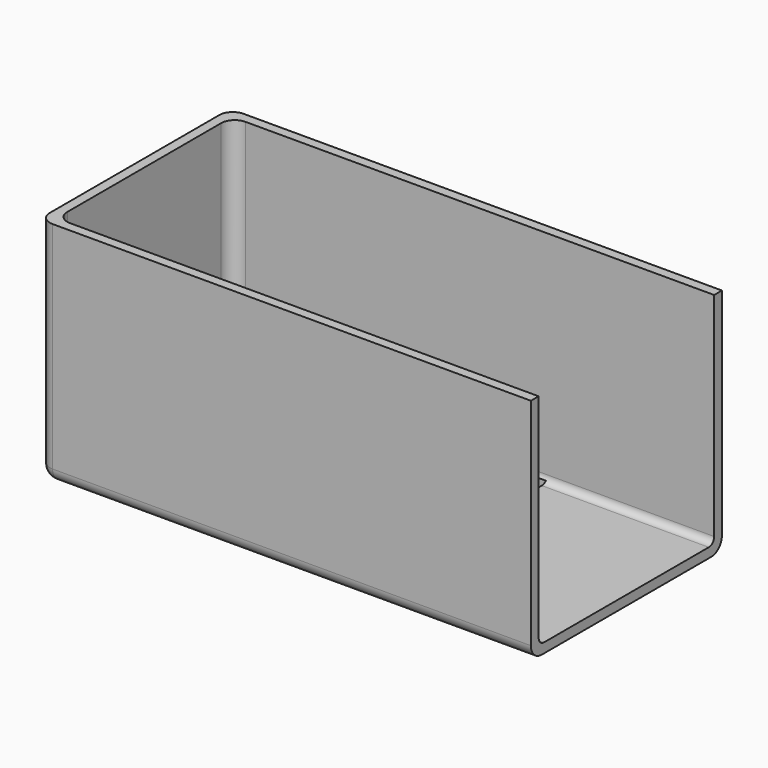
from build123d import *

# Parameters (mm, degrees)
F0_W         = 74.44
F0_H         = 35.44
F1_DEPTH     = 34
F2_T         = -1.44
F3_DEPTH     = 1.44
F4_R         = 2
F5_R         = 2
F6_W         = 22
F6_H         = 2
F7_DEPTH     = 1.441
F8_T1_DEPTH  = 28.56
F8_T6_DEPTH  = 69.56
F8_T12_DEPTH = 69.56
F8_T18_DEPTH = 69.56
F8_T25_DEPTH = 69.56
F8_T31_DEPTH = 69.56
F8_T35_ANGLE = 90
F8_T37_ANGLE = 90
F8_T41_DEPTH = 69.56
F8_T47_DEPTH = 69.56
F8_T53_DEPTH = 69.56
F8_T60_DEPTH = 69.56
F8_T66_DEPTH = 69.56


# Not quite as in the source:
# - a fillet or chamfer that OpenCascade refuses, or shapes differently, is made with other operations: its cross-section is extruded or revolved along the edge and cut away or added


with BuildPart() as f1:
    # F0 (on Top) → F1 (new body)
    with BuildSketch(Plane.XY):
        Rectangle(F0_W, F0_H)
    extrude(amount=F1_DEPTH)

    # F2
    f2_openings = [f1.faces().sort_by_distance(p)[0] for p in [
        (0, 0, 34),
    ]]
    offset(amount=F2_T, openings=f2_openings)

    # F3 (cut): a face of the model
    f3_faces = [f1.faces().sort_by_distance(p)[0] for p in [
        (37.22, 0, 17),
    ]]
    extrude(f3_faces, amount=-F3_DEPTH, mode=Mode.SUBTRACT)

    # F4
    f4_edges = [f1.edges().sort_by_distance(p)[0] for p in [
        (-35.78, -16.28, 17.72),
        (-35.78, 16.28, 17.72),
        (-37.22, 17.72, 17),
        (-37.22, -17.72, 17),
    ]]
    fillet(f4_edges, radius=F4_R)

    # F5
    f5_edges = [f1.edges().sort_by_distance(p)[0] for p in [
        (-37.22, 0, 0),
        (0.28, -17.72, 0),
        (0.28, 17.72, 0),
    ]]
    fillet(f5_edges, radius=F5_R)

    # F6 (on face) → F7 (cut, through all)
    with BuildSketch(Plane.XY.offset(1.44)):
        with Locations((0, 15.03)):
            Rectangle(F6_W, F6_H)
        with Locations((0, -15.03)):
            Rectangle(F6_W, F6_H)
    extrude(amount=-F7_DEPTH, mode=Mode.SUBTRACT)

    # F8: fillet of radius 1 on 1 edges, made by hand

    # F8_s2 → F8_t1 (join)
    with BuildSketch(Plane.XZ.offset(-14.28)):
        with BuildLine():
            ThreePointArc((-35.78, 2.44), (-35.4871067812, 1.7328932188), (-34.78, 1.44))
            Line((-34.78, 1.44), (-35.78, 1.44))
            Line((-35.78, 1.44), (-35.78, 2.44))
        make_face()
    extrude(amount=F8_T1_DEPTH)


with BuildPart() as f8_tool4:
    # F8_s5 → F8_t6 (new body)
    with BuildSketch(Plane.YZ.offset(-33.78)):
        with BuildLine():
            ThreePointArc((-16.28, 2.44), (-15.9871067812, 1.7328932188), (-15.28, 1.44))
            Line((-15.28, 1.44), (-16.28, 1.44))
            Line((-16.28, 1.44), (-16.28, 2.44))
        make_face()
    extrude(amount=F8_T6_DEPTH)

    split(bisect_by=Plane.YZ.offset(-11), keep=Keep.BOTTOM)

    split(bisect_by=Plane.XZ.offset(16.03), keep=Keep.TOP)


with BuildPart() as f1_1:
    add(f1.part)

    # F8_t3: union F8_tool4
    add(f8_tool4.part)


with BuildPart() as f8_tool10:
    # F8_s11 → F8_t12 (new body)
    with BuildSketch(Plane.YZ.offset(-33.78)):
        with BuildLine():
            ThreePointArc((-16.28, 2.44), (-15.9871067812, 1.7328932188), (-15.28, 1.44))
            Line((-15.28, 1.44), (-16.28, 1.44))
            Line((-16.28, 1.44), (-16.28, 2.44))
        make_face()
    extrude(amount=F8_T12_DEPTH)

    split(bisect_by=Plane.YZ.offset(-11), keep=Keep.BOTTOM)

    split(bisect_by=Plane.XZ.offset(16.03), keep=Keep.BOTTOM)


with BuildPart() as f1_2:
    add(f1_1.part)

    # F8_t9: union F8_tool10
    add(f8_tool10.part)


with BuildPart() as f8_tool16:
    # F8_s17 → F8_t18 (new body)
    with BuildSketch(Plane.YZ.offset(-33.78)):
        with BuildLine():
            ThreePointArc((-16.28, 2.44), (-15.9871067812, 1.7328932188), (-15.28, 1.44))
            Line((-15.28, 1.44), (-16.28, 1.44))
            Line((-16.28, 1.44), (-16.28, 2.44))
        make_face()
    extrude(amount=F8_T18_DEPTH)

    split(bisect_by=Plane.YZ.offset(-11), keep=Keep.TOP)

    split(bisect_by=Plane.XZ.offset(16.03), keep=Keep.TOP)

    split(bisect_by=Plane.YZ.offset(11), keep=Keep.BOTTOM)


with BuildPart() as f1_3:
    add(f1_2.part)

    # F8_t15: union F8_tool16
    add(f8_tool16.part)


with BuildPart() as f8_tool23:
    # F8_s24 → F8_t25 (new body)
    with BuildSketch(Plane.YZ.offset(-33.78)):
        with BuildLine():
            ThreePointArc((-16.28, 2.44), (-15.9871067812, 1.7328932188), (-15.28, 1.44))
            Line((-15.28, 1.44), (-16.28, 1.44))
            Line((-16.28, 1.44), (-16.28, 2.44))
        make_face()
    extrude(amount=F8_T25_DEPTH)

    split(bisect_by=Plane.XZ.offset(16.03), keep=Keep.TOP)

    split(bisect_by=Plane.YZ.offset(11), keep=Keep.TOP)


with BuildPart() as f1_4:
    add(f1_3.part)

    # F8_t22: union F8_tool23
    add(f8_tool23.part)


with BuildPart() as f8_tool29:
    # F8_s30 → F8_t31 (new body)
    with BuildSketch(Plane.YZ.offset(-33.78)):
        with BuildLine():
            ThreePointArc((-16.28, 2.44), (-15.9871067812, 1.7328932188), (-15.28, 1.44))
            Line((-15.28, 1.44), (-16.28, 1.44))
            Line((-16.28, 1.44), (-16.28, 2.44))
        make_face()
    extrude(amount=F8_T31_DEPTH)

    split(bisect_by=Plane.XZ.offset(16.03), keep=Keep.BOTTOM)

    split(bisect_by=Plane.YZ.offset(11), keep=Keep.TOP)


with BuildPart() as f1_5:
    add(f1_4.part)

    # F8_t28: union F8_tool29
    add(f8_tool29.part)

    # F8_s34 → F8_t35 (revolve)
    with BuildSketch(Plane.XZ.offset(14.28)):
        with BuildLine():
            ThreePointArc((-35.78, 2.44), (-35.4871067812, 1.7328932188), (-34.78, 1.44))
            Line((-34.78, 1.44), (-35.78, 1.44))
            Line((-35.78, 1.44), (-35.78, 2.44))
        make_face()
    revolve(axis=Axis((-33.78, -14.28, 1.44), (0, 0, 1)), revolution_arc=F8_T35_ANGLE)

    # F8_s36 → F8_t37 (revolve)
    with BuildSketch(Plane.YZ.offset(-33.78)):
        with BuildLine():
            ThreePointArc((16.28, 2.44), (15.9871067812, 1.7328932188), (15.28, 1.44))
            Line((15.28, 1.44), (16.28, 1.44))
            Line((16.28, 1.44), (16.28, 2.44))
        make_face()
    revolve(axis=Axis((-33.78, 14.28, 1.44), (0, 0, 1)), revolution_arc=F8_T37_ANGLE)


with BuildPart() as f8_tool39:
    # F8_s40 → F8_t41 (new body)
    with BuildSketch(Plane.YZ.offset(35.78)):
        with BuildLine():
            ThreePointArc((16.28, 2.44), (15.9871067812, 1.7328932188), (15.28, 1.44))
            Line((15.28, 1.44), (16.28, 1.44))
            Line((16.28, 1.44), (16.28, 2.44))
        make_face()
    extrude(amount=-F8_T41_DEPTH)

    split(bisect_by=Plane.YZ.offset(11), keep=Keep.TOP)

    split(bisect_by=Plane.XZ.offset(-16.03), keep=Keep.BOTTOM)


with BuildPart() as f1_6:
    add(f1_5.part)

    # F8_t38: union F8_tool39
    add(f8_tool39.part)


with BuildPart() as f8_tool45:
    # F8_s46 → F8_t47 (new body)
    with BuildSketch(Plane.YZ.offset(35.78)):
        with BuildLine():
            ThreePointArc((16.28, 2.44), (15.9871067812, 1.7328932188), (15.28, 1.44))
            Line((15.28, 1.44), (16.28, 1.44))
            Line((16.28, 1.44), (16.28, 2.44))
        make_face()
    extrude(amount=-F8_T47_DEPTH)

    split(bisect_by=Plane.YZ.offset(11), keep=Keep.TOP)

    split(bisect_by=Plane.XZ.offset(-16.03), keep=Keep.TOP)


with BuildPart() as f1_7:
    add(f1_6.part)

    # F8_t44: union F8_tool45
    add(f8_tool45.part)


with BuildPart() as f8_tool51:
    # F8_s52 → F8_t53 (new body)
    with BuildSketch(Plane.YZ.offset(35.78)):
        with BuildLine():
            ThreePointArc((16.28, 2.44), (15.9871067812, 1.7328932188), (15.28, 1.44))
            Line((15.28, 1.44), (16.28, 1.44))
            Line((16.28, 1.44), (16.28, 2.44))
        make_face()
    extrude(amount=-F8_T53_DEPTH)

    split(bisect_by=Plane.YZ.offset(11), keep=Keep.BOTTOM)

    split(bisect_by=Plane.XZ.offset(-16.03), keep=Keep.BOTTOM)

    split(bisect_by=Plane.YZ.offset(-11), keep=Keep.TOP)


with BuildPart() as f1_8:
    add(f1_7.part)

    # F8_t50: union F8_tool51
    add(f8_tool51.part)


with BuildPart() as f8_tool58:
    # F8_s59 → F8_t60 (new body)
    with BuildSketch(Plane.YZ.offset(35.78)):
        with BuildLine():
            ThreePointArc((16.28, 2.44), (15.9871067812, 1.7328932188), (15.28, 1.44))
            Line((15.28, 1.44), (16.28, 1.44))
            Line((16.28, 1.44), (16.28, 2.44))
        make_face()
    extrude(amount=-F8_T60_DEPTH)

    split(bisect_by=Plane.XZ.offset(-16.03), keep=Keep.BOTTOM)

    split(bisect_by=Plane.YZ.offset(-11), keep=Keep.BOTTOM)


with BuildPart() as f1_9:
    add(f1_8.part)

    # F8_t57: union F8_tool58
    add(f8_tool58.part)


with BuildPart() as f8_tool64:
    # F8_s65 → F8_t66 (new body)
    with BuildSketch(Plane.YZ.offset(35.78)):
        with BuildLine():
            ThreePointArc((16.28, 2.44), (15.9871067812, 1.7328932188), (15.28, 1.44))
            Line((15.28, 1.44), (16.28, 1.44))
            Line((16.28, 1.44), (16.28, 2.44))
        make_face()
    extrude(amount=-F8_T66_DEPTH)

    split(bisect_by=Plane.XZ.offset(-16.03), keep=Keep.TOP)

    split(bisect_by=Plane.YZ.offset(-11), keep=Keep.BOTTOM)


with BuildPart() as f1_10:
    add(f1_9.part)

    # F8_t63: union F8_tool64
    add(f8_tool64.part)


solid = f1_10.part
